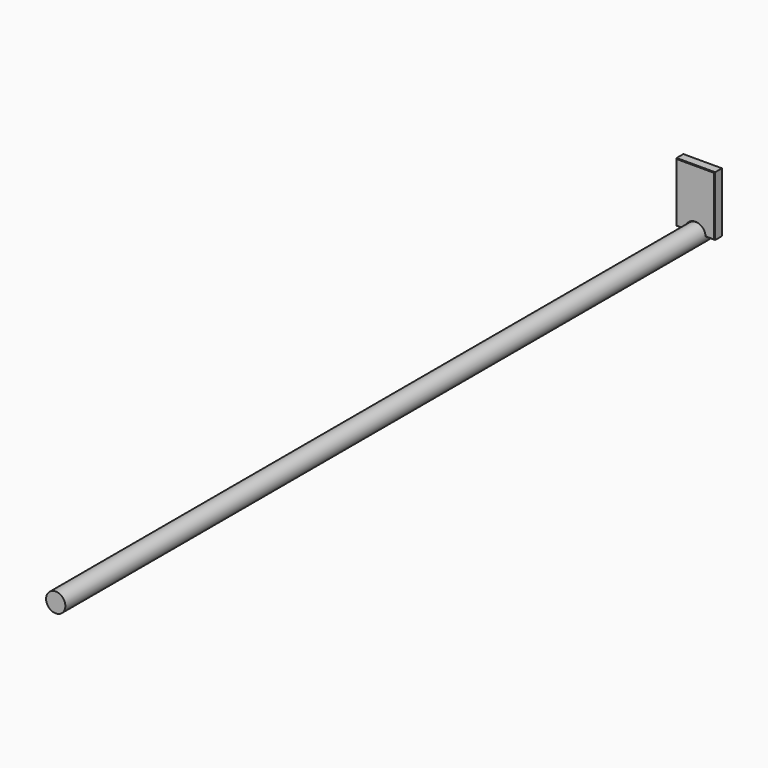
from build123d import *

# Parameters (mm, degrees)
F0_R         = 5
F1_DEPTH     = 400
F2_TEXT_SIZE = 6.3287186427
F3_DEPTH     = 5
F4_SIZE      = 0.3
F5_DEPTH     = 0.5
F6_DEPTH     = 420


# Not quite as in the source:
# - Text() gives the source's letters only with a copy of the font that has no kerning and outlines rounded to 1/6400 em; it was checked with that copy


with BuildPart() as f1:
    # F0 (on Front) → F1 (new body)
    with BuildSketch(Plane.XZ):
        Circle(F0_R)
    extrude(amount=F1_DEPTH)


with BuildPart() as f3:
    # F2 (on Front) → F3 (new body)
    with BuildSketch(Plane.XZ):
        with BuildLine():
            Line((10, 31), (-10, 31))
            Line((-10, 31), (-10, 0))
            Line((-10, 0), (-5, 0))
            ThreePointArc((-5, 0), (0, 5), (5, 0))
            Line((5, 0), (10, 0))
            Line((10, 0), (10, 31))
        make_face()
        with BuildLine():
            add(Edge.make_bspline(
                [(-2.0197512231, 13.8291350057), (-1.7354533153, 14.2355574061), (-1.2291558239, 14.2355574061)],
                knots=[0, 0, 0, 1, 1, 1], degree=2))
            add(Edge.make_bspline(
                [(-1.2291558239, 14.2355574061), (-0.8059227647, 14.2355574061), (-0.5092640783, 13.9789476423)],
                knots=[0, 0, 0, 1, 1, 1], degree=2))
            add(Edge.make_bspline(
                [(-0.5092640783, 13.9789476423), (-0.2126053919, 13.7223378786), (-0.1008639534, 13.2585614656)],
                knots=[0, 0, 0, 1, 1, 1], degree=2))
            Line((-0.1008639534, 13.2585614656), (-0.0830644322, 13.2585614656))
            add(Edge.make_bspline(
                [(-0.0830644322, 13.2585614656), (-0.0148329343, 13.8063911731), (0.2496877277, 14.0872280629)],
                knots=[0, 0, 0, 1, 1, 1], degree=2))
            add(Edge.make_bspline(
                [(0.2496877277, 14.0872280629), (0.5142083897, 14.3680649526), (0.9621630061, 14.3680649526)],
                knots=[0, 0, 0, 1, 1, 1], degree=2))
            add(Edge.make_bspline(
                [(0.9621630061, 14.3680649526), (1.6138232539, 14.3680649526), (1.9772301447, 13.895388779)],
                knots=[0, 0, 0, 1, 1, 1], degree=2))
            add(Edge.make_bspline(
                [(1.9772301447, 13.895388779), (2.3406370355, 13.4227126054), (2.3406370355, 12.545591756)],
                knots=[0, 0, 0, 1, 1, 1], degree=2))
            add(Edge.make_bspline(
                [(2.3406370355, 12.545591756), (2.3406370355, 11.8098782138), (2.0963880504, 11.2412823983)],
                knots=[0, 0, 0, 1, 1, 1], degree=2))
            Line((2.0963880504, 11.2412823983), (1.2835432497, 11.2412823983))
            add(Edge.make_bspline(
                [(1.2835432497, 11.2412823983), (1.4160507963, 11.5033309045), (1.4996096596, 11.8187779744)],
                knots=[0, 0, 0, 1, 1, 1], degree=2))
            add(Edge.make_bspline(
                [(1.4996096596, 11.8187779744), (1.583168523, 12.1342250442), (1.583168523, 12.4427500781)],
                knots=[0, 0, 0, 1, 1, 1], degree=2))
            add(Edge.make_bspline(
                [(1.583168523, 12.4427500781), (1.583168523, 12.916415114), (1.4224784012, 13.1418757156)],
                knots=[0, 0, 0, 1, 1, 1], degree=2))
            add(Edge.make_bspline(
                [(1.4224784012, 13.1418757156), (1.2617882794, 13.3673363173), (0.9057978557, 13.3673363173)],
                knots=[0, 0, 0, 1, 1, 1], degree=2))
            add(Edge.make_bspline(
                [(0.9057978557, 13.3673363173), (0.5883730613, 13.3673363173), (0.4553710836, 13.1077599667)],
                knots=[0, 0, 0, 1, 1, 1], degree=2))
            add(Edge.make_bspline(
                [(0.4553710836, 13.1077599667), (0.3223691059, 12.8481836161), (0.3223691059, 12.2795878006)],
                knots=[0, 0, 0, 1, 1, 1], degree=2))
            Line((0.3223691059, 12.2795878006), (0.3223691059, 11.9364525867))
            Line((0.3223691059, 11.9364525867), (-0.4103778495, 11.9364525867))
            Line((-0.4103778495, 11.9364525867), (-0.4103778495, 12.2855209743))
            add(Edge.make_bspline(
                [(-0.4103778495, 12.2855209743), (-0.4103778495, 12.8106068492), (-0.5478297075, 13.0533725409)],
                knots=[0, 0, 0, 1, 1, 1], degree=2))
            add(Edge.make_bspline(
                [(-0.5478297075, 13.0533725409), (-0.6852815655, 13.2961382325), (-1.0185281566, 13.2961382325)],
                knots=[0, 0, 0, 1, 1, 1], degree=2))
            add(Edge.make_bspline(
                [(-1.0185281566, 13.2961382325), (-1.531747684, 13.2961382325), (-1.531747684, 12.6533777454)],
                knots=[0, 0, 0, 1, 1, 1], degree=2))
            add(Edge.make_bspline(
                [(-1.531747684, 12.6533777454), (-1.531747684, 12.4308837306), (-1.4575830124, 12.2004788175)],
                knots=[0, 0, 0, 1, 1, 1], degree=2))
            add(Edge.make_bspline(
                [(-1.4575830124, 12.2004788175), (-1.3834183408, 11.9700739044), (-1.2014676798, 11.6892370147)],
                knots=[0, 0, 0, 1, 1, 1], degree=2))
            Line((-1.2014676798, 11.6892370147), (-1.8590611013, 11.247215572))
            add(Edge.make_bspline(
                [(-1.8590611013, 11.247215572), (-2.3040491308, 11.8652545019), (-2.3040491308, 12.7216092433)],
                knots=[0, 0, 0, 1, 1, 1], degree=2))
            add(Edge.make_bspline(
                [(-2.3040491308, 12.7216092433), (-2.3040491308, 13.4227126054), (-2.0197512231, 13.8291350057)],
                knots=[0, 0, 0, 1, 1, 1], degree=2))
        make_face(mode=Mode.SUBTRACT)
        with BuildLine():
            Line((-2.2397730821, 17.226865827), (2.2783387114, 17.226865827))
            Line((2.2783387114, 17.226865827), (2.2783387114, 16.2716248569))
            Line((2.2783387114, 16.2716248569), (-0.3362131779, 16.2716248569))
            Line((-0.3362131779, 16.2716248569), (-0.7653794108, 16.2815134798))
            Line((-0.7653794108, 16.2815134798), (-1.2350889976, 16.2963464141))
            add(Edge.make_bspline(
                [(-1.2350889976, 16.2963464141), (-0.9977620485, 16.059019465), (-0.9235973769, 15.9660664099)],
                knots=[0, 0, 0, 1, 1, 1], degree=2))
            Line((-0.9235973769, 15.9660664099), (-0.5062974914, 15.4469137088))
            Line((-0.5062974914, 15.4469137088), (-1.0808264807, 14.9861038826))
            Line((-1.0808264807, 14.9861038826), (-2.2397730821, 16.4417091704))
            Line((-2.2397730821, 16.4417091704), (-2.2397730821, 17.226865827))
        make_face(mode=Mode.SUBTRACT)
        with BuildLine():
            Line((2.2783387114, 21.5837930676), (2.2783387114, 20.7056833559))
            Line((2.2783387114, 20.7056833559), (-1.2657437285, 19.6179348392))
            Line((-1.2657437285, 19.6179348392), (-1.2657437285, 19.5902466951))
            add(Edge.make_bspline(
                [(-1.2657437285, 19.5902466951), (-0.1849172478, 19.6495784324), (0.1770063495, 19.6495784324)],
                knots=[0, 0, 0, 1, 1, 1], degree=2))
            Line((0.1770063495, 19.6495784324), (2.2783387114, 19.6495784324))
            Line((2.2783387114, 19.6495784324), (2.2783387114, 18.7932236911))
            Line((2.2783387114, 18.7932236911), (-2.2397730821, 18.7932236911))
            Line((-2.2397730821, 18.7932236911), (-2.2397730821, 20.0975330488))
            Line((-2.2397730821, 20.0975330488), (1.2153117518, 21.1664931821))
            Line((1.2153117518, 21.1664931821), (1.2153117518, 21.1852815655))
            Line((1.2153117518, 21.1852815655), (-2.2397730821, 22.3195066098))
            Line((-2.2397730821, 22.3195066098), (-2.2397730821, 23.6228271052))
            Line((-2.2397730821, 23.6228271052), (2.2783387114, 23.6228271052))
            Line((2.2783387114, 23.6228271052), (2.2783387114, 22.7298844592))
            Line((2.2783387114, 22.7298844592), (0.1394295826, 22.7298844592))
            add(Edge.make_bspline(
                [(0.1394295826, 22.7298844592), (-0.0118663475, 22.7298844592), (-0.209638805, 22.7348287707)],
                knots=[0, 0, 0, 1, 1, 1], degree=2))
            add(Edge.make_bspline(
                [(-0.209638805, 22.7348287707), (-0.4074112626, 22.7397730821), (-1.2598105548, 22.7763609868)],
                knots=[0, 0, 0, 1, 1, 1], degree=2))
            Line((-1.2598105548, 22.7763609868), (-1.2598105548, 22.7486728427))
            Line((-1.2598105548, 22.7486728427), (2.2783387114, 21.5837930676))
        make_face(mode=Mode.SUBTRACT)
        with BuildLine():
            Line((2.2783387114, 27.5505881128), (2.2783387114, 26.6724784012))
            Line((2.2783387114, 26.6724784012), (-1.2657437285, 25.5847298845))
            Line((-1.2657437285, 25.5847298845), (-1.2657437285, 25.5570417404))
            add(Edge.make_bspline(
                [(-1.2657437285, 25.5570417404), (-0.1849172478, 25.6163734777), (0.1770063495, 25.6163734777)],
                knots=[0, 0, 0, 1, 1, 1], degree=2))
            Line((0.1770063495, 25.6163734777), (2.2783387114, 25.6163734777))
            Line((2.2783387114, 25.6163734777), (2.2783387114, 24.7600187363))
            Line((2.2783387114, 24.7600187363), (-2.2397730821, 24.7600187363))
            Line((-2.2397730821, 24.7600187363), (-2.2397730821, 26.0643280941))
            Line((-2.2397730821, 26.0643280941), (1.2153117518, 27.1332882273))
            Line((1.2153117518, 27.1332882273), (1.2153117518, 27.1520766108))
            Line((1.2153117518, 27.1520766108), (-2.2397730821, 28.286301655))
            Line((-2.2397730821, 28.286301655), (-2.2397730821, 29.5896221505))
            Line((-2.2397730821, 29.5896221505), (2.2783387114, 29.5896221505))
            Line((2.2783387114, 29.5896221505), (2.2783387114, 28.6966795045))
            Line((2.2783387114, 28.6966795045), (0.1394295826, 28.6966795045))
            add(Edge.make_bspline(
                [(0.1394295826, 28.6966795045), (-0.0118663475, 28.6966795045), (-0.209638805, 28.701623816)],
                knots=[0, 0, 0, 1, 1, 1], degree=2))
            add(Edge.make_bspline(
                [(-0.209638805, 28.701623816), (-0.4074112626, 28.7065681274), (-1.2598105548, 28.7431560321)],
                knots=[0, 0, 0, 1, 1, 1], degree=2))
            Line((-1.2598105548, 28.7431560321), (-1.2598105548, 28.715467888))
            Line((-1.2598105548, 28.715467888), (2.2783387114, 27.5505881128))
        make_face(mode=Mode.SUBTRACT)
        with Locations(Location((2.2783387114, 11), (0, 0, 90))):
            Text('31MM', F2_TEXT_SIZE, font='Open Sans', font_style=FontStyle.BOLD, text_align=(TextAlign.LEFT, TextAlign.BOTTOM))
    extrude(amount=F3_DEPTH)

    # F4
    f4_edges = [f3.edges().sort_by_distance(p)[0] for p in [
        (0, -5, 31),
        (10, -5, 15.5),
        (7.5, -5, 0),
        (0, -5, 5),
        (-7.5, -5, 0),
        (-10, -5, 15.5),
        (0, 0, 31),
        (10, 0, 15.5),
        (7.5, 0, 0),
        (0, 0, 5),
        (-7.5, 0, 0),
        (-10, 0, 15.5),
    ]]
    chamfer(f4_edges, length=F4_SIZE)

    # F2 (on Front) → F5 (cut)
    with BuildSketch(Plane.XZ):
        with Locations(Location((2.2783387114, 11), (0, 0, 90))):
            Text('31MM', F2_TEXT_SIZE, font='Open Sans', font_style=FontStyle.BOLD, text_align=(TextAlign.LEFT, TextAlign.BOTTOM))
    extrude(amount=F5_DEPTH, mode=Mode.SUBTRACT)


with BuildPart() as f6:
    # F0 (on Front) → F6 (new body)
    with BuildSketch(Plane.XZ):
        Circle(F0_R)
    extrude(amount=F6_DEPTH)


solid = Compound([f1.part, f3.part, f6.part])
